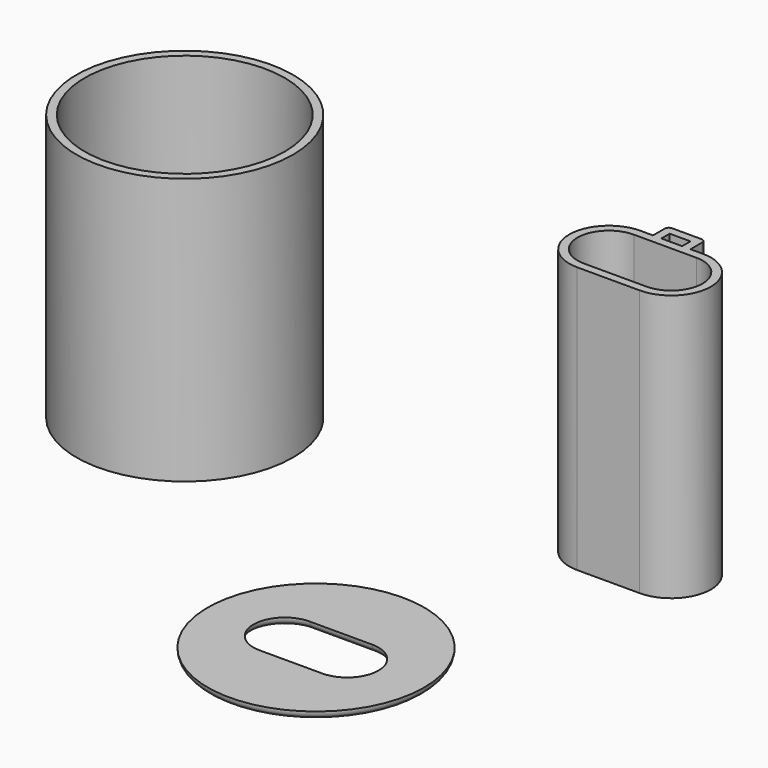
from build123d import *

# Parameters (mm, degrees)
F0_R         = 33.02
F0_R_2       = 30.48
F1_DEPTH     = 81.28
F2_DEPTH     = 2.54
F3_DEPTH     = 1.27
F4_T1_DEPTH  = 19.05
F4_T8_ANGLE  = 180
F4_T12_ANGLE = 180


# Not quite as in the source:
# - a fillet or chamfer that OpenCascade refuses, or shapes differently, is made with other operations: its cross-section is extruded or revolved along the edge and cut away or added


with BuildPart() as f1:
    # F0 (on Top) → F1 (new body)
    with BuildSketch(Plane.XY):
        with Locations((-97.8379249573, 24.8728301376)):
            Circle(F0_R)
        with Locations((-97.8379249573, 24.8728301376)):
            Circle(F0_R_2, mode=Mode.SUBTRACT)
    extrude(amount=F1_DEPTH)


with BuildPart() as f1b:
    # F0 (on Top) → F1, piece 2 (new body)
    with BuildSketch(Plane.XY):
        with BuildLine():
            Line((36.9737733483, 45.9476387101), (39.5137733483, 45.9476387101))
            Line((39.5137733483, 45.9476387101), (39.5137733483, 50.3926387101))
            ThreePointArc((39.5137733483, 50.3926387101), (39.1417989604, 51.2906643222), (38.2437733483, 51.6626387101))
            Line((38.2437733483, 51.6626387101), (29.3537733483, 51.6626387101))
            ThreePointArc((29.3537733483, 51.6626387101), (28.4557477362, 51.2906643222), (28.0837733483, 50.3926387101))
            Line((28.0837733483, 50.3926387101), (28.0837733483, 45.9476387101))
            Line((28.0837733483, 45.9476387101), (30.6237733483, 45.9476387101))
            Line((30.6237733483, 45.9476387101), (30.6237733483, 49.1226387101))
            Line((30.6237733483, 49.1226387101), (36.9737733483, 49.1226387101))
            Line((36.9737733483, 49.1226387101), (36.9737733483, 45.9476387101))
        make_face()
        with BuildLine():
            ThreePointArc((43.3237733483, 21.8176387101), (55.3887733483, 33.8826387101), (43.3237733483, 45.9476387101))
            Line((43.3237733483, 45.9476387101), (39.5137733483, 45.9476387101))
            Line((39.5137733483, 45.9476387101), (36.9737733483, 45.9476387101))
            Line((36.9737733483, 45.9476387101), (30.6237733483, 45.9476387101))
            Line((30.6237733483, 45.9476387101), (28.0837733483, 45.9476387101))
            Line((28.0837733483, 45.9476387101), (24.2737733483, 45.9476387101))
            ThreePointArc((24.2737733483, 45.9476387101), (12.2087733483, 33.8826387101), (24.2737733483, 21.8176387101))
            Line((24.2737733483, 21.8176387101), (43.3237733483, 21.8176387101))
        make_face()
        with BuildLine():
            ThreePointArc((24.2737733483, 24.3576387101), (14.7487733483, 33.8826387101), (24.2737733483, 43.4076387101))
            Line((24.2737733483, 43.4076387101), (43.3237733483, 43.4076387101))
            ThreePointArc((43.3237733483, 43.4076387101), (52.8487733483, 33.8826387101), (43.3237733483, 24.3576387101))
            Line((43.3237733483, 24.3576387101), (24.2737733483, 24.3576387101))
        make_face(mode=Mode.SUBTRACT)
    extrude(amount=F1_DEPTH)


with BuildPart() as f2:
    # F0 (on Top) → F2 (new body)
    with BuildSketch(Plane.XY):
        with BuildLine():
            Line((23.8957638139, -31.8045213862), (27.0388534563, -28.6614317439))
            ThreePointArc((27.0388534563, -28.6614317439), (-19.6584783733, -28.6614317439), (-19.6584783733, -75.3587635734))
            Line((-19.6584783733, -75.3587635734), (-16.5153887309, -72.215673931))
            ThreePointArc((-16.5153887309, -72.215673931), (-16.5153887309, -67.7255458705), (-12.0252606704, -67.7255458705))
            Line((-12.0252606704, -67.7255458705), (-5.8348124585, -61.5350976586))
            ThreePointArc((-5.8348124585, -61.5350976586), (-15.3598124585, -52.0100976586), (-5.8348124585, -42.4850976586))
            Line((-5.8348124585, -42.4850976586), (13.2151875415, -42.4850976586))
            Line((13.2151875415, -42.4850976586), (19.4056357534, -36.2946494468))
            ThreePointArc((19.4056357534, -36.2946494468), (19.4056357534, -31.8045213862), (23.8957638139, -31.8045213862))
        make_face()
        with BuildLine():
            ThreePointArc((-19.6584783733, -75.3587635734), (16.3263944782, -82.5165998222), (36.7101875415, -52.0100976586))
            ThreePointArc((36.7101875415, -52.0100976586), (34.196689705, -39.3738907219), (27.0388534563, -28.6614317439))
            Line((27.0388534563, -28.6614317439), (23.8957638139, -31.8045213862))
            ThreePointArc((23.8957638139, -31.8045213862), (24.5840172994, -32.8345655187), (24.8256997837, -34.0495854165))
            ThreePointArc((24.8256997837, -34.0495854165), (22.8657196814, -36.9829029322), (19.4056357534, -36.2946494468))
            Line((19.4056357534, -36.2946494468), (13.2151875415, -42.4850976586))
            ThreePointArc((13.2151875415, -42.4850976586), (22.7401875415, -52.0100976586), (13.2151875415, -61.5350976586))
            Line((13.2151875415, -61.5350976586), (-5.8348124585, -61.5350976586))
            Line((-5.8348124585, -61.5350976586), (-12.0252606704, -67.7255458705))
            ThreePointArc((-12.0252606704, -67.7255458705), (-11.3370071849, -68.755590003), (-11.0953247006, -69.9706099008))
            ThreePointArc((-11.0953247006, -69.9706099008), (-13.0553048029, -72.9039274165), (-16.5153887309, -72.215673931))
            Line((-16.5153887309, -72.215673931), (-19.6584783733, -75.3587635734))
        make_face()
        with BuildLine():
            Line((-14.2703247006, -69.9706099008), (-16.5153887309, -72.215673931))
            ThreePointArc((-16.5153887309, -72.215673931), (-13.0553048029, -72.9039274165), (-11.0953247006, -69.9706099008))
            ThreePointArc((-11.0953247006, -69.9706099008), (-11.3370071849, -68.755590003), (-12.0252606704, -67.7255458705))
            Line((-12.0252606704, -67.7255458705), (-14.2703247006, -69.9706099008))
        make_face()
        with BuildLine():
            ThreePointArc((-12.0252606704, -67.7255458705), (-16.5153887309, -67.7255458705), (-16.5153887309, -72.215673931))
            Line((-16.5153887309, -72.215673931), (-14.2703247006, -69.9706099008))
            Line((-14.2703247006, -69.9706099008), (-12.0252606704, -67.7255458705))
        make_face()
        with BuildLine():
            Line((21.6506997837, -34.0495854165), (23.8957638139, -31.8045213862))
            ThreePointArc((23.8957638139, -31.8045213862), (19.4056357534, -31.8045213862), (19.4056357534, -36.2946494468))
            Line((19.4056357534, -36.2946494468), (21.6506997837, -34.0495854165))
        make_face()
        with BuildLine():
            ThreePointArc((24.8256997837, -34.0495854165), (24.5840172994, -32.8345655187), (23.8957638139, -31.8045213862))
            Line((23.8957638139, -31.8045213862), (21.6506997837, -34.0495854165))
            Line((21.6506997837, -34.0495854165), (19.4056357534, -36.2946494468))
            ThreePointArc((19.4056357534, -36.2946494468), (22.8657196814, -36.9829029322), (24.8256997837, -34.0495854165))
        make_face()
    extrude(amount=F2_DEPTH)

    # F0 (on Top) → F3 (join)
    with BuildSketch(Plane.XY):
        with BuildLine():
            ThreePointArc((24.8256997837, -34.0495854165), (24.5840172994, -32.8345655187), (23.8957638139, -31.8045213862))
            Line((23.8957638139, -31.8045213862), (21.6506997837, -34.0495854165))
            Line((21.6506997837, -34.0495854165), (19.4056357534, -36.2946494468))
            ThreePointArc((19.4056357534, -36.2946494468), (22.8657196814, -36.9829029322), (24.8256997837, -34.0495854165))
        make_face()
        with BuildLine():
            Line((21.6506997837, -34.0495854165), (23.8957638139, -31.8045213862))
            ThreePointArc((23.8957638139, -31.8045213862), (19.4056357534, -31.8045213862), (19.4056357534, -36.2946494468))
            Line((19.4056357534, -36.2946494468), (21.6506997837, -34.0495854165))
        make_face()
        with BuildLine():
            ThreePointArc((-12.0252606704, -67.7255458705), (-16.5153887309, -67.7255458705), (-16.5153887309, -72.215673931))
            Line((-16.5153887309, -72.215673931), (-14.2703247006, -69.9706099008))
            Line((-14.2703247006, -69.9706099008), (-12.0252606704, -67.7255458705))
        make_face()
        with BuildLine():
            Line((-14.2703247006, -69.9706099008), (-16.5153887309, -72.215673931))
            ThreePointArc((-16.5153887309, -72.215673931), (-13.0553048029, -72.9039274165), (-11.0953247006, -69.9706099008))
            ThreePointArc((-11.0953247006, -69.9706099008), (-11.3370071849, -68.755590003), (-12.0252606704, -67.7255458705))
            Line((-12.0252606704, -67.7255458705), (-14.2703247006, -69.9706099008))
        make_face()
    extrude(amount=-F3_DEPTH)

    # F4: fillet of radius 2.54 on 7 edges, made by hand

    # F4_s2 → F4_t1 (cut)
    with BuildSketch(Plane.YZ.offset(-5.8348124585)):
        with BuildLine():
            ThreePointArc((-64.0750976586, 0), (-62.2790464344, 0.7439487758), (-61.5350976586, 2.54))
            Line((-61.5350976586, 2.54), (-61.5350976586, 0))
            Line((-61.5350976586, 0), (-64.0750976586, 0))
        make_face()
        with BuildLine():
            ThreePointArc((-39.9450976586, 0), (-41.7411488828, 0.7439487758), (-42.4850976586, 2.54))
            Line((-42.4850976586, 2.54), (-42.4850976586, 0))
            Line((-42.4850976586, 0), (-39.9450976586, 0))
        make_face()
    extrude(amount=F4_T1_DEPTH, mode=Mode.SUBTRACT)

    # F4_s3 → F4_t4 (revolve, cut)
    with BuildSketch(Plane.XZ.offset(34.0495854165)):
        with BuildLine():
            ThreePointArc((24.8256997837, 0), (23.895995258, -0.9297045256), (22.625995258, -1.27))
            Line((22.625995258, -1.27), (24.8256997837, -1.27))
            Line((24.8256997837, -1.27), (24.8256997837, 0))
        make_face()
    revolve(axis=Axis((21.6506997837, -34.0495854165, -1.27), (0, 0, 1)), mode=Mode.SUBTRACT)

    # F4_s5 → F4_t6 (revolve, cut)
    with BuildSketch(Plane(origin=(27.8501426001, -27.8501426001, 0), x_dir=(0, 0, 1), z_dir=(-0.7071067812, 0.7071067812, 0))):
        with BuildLine():
            ThreePointArc((0, -62.7423361101), (-0.9297045256, -61.8126315845), (-1.27, -60.5426315845))
            Line((-1.27, -60.5426315845), (-1.27, -62.7423361101))
            Line((-1.27, -62.7423361101), (0, -62.7423361101))
        make_face()
    revolve(axis=Axis((-14.2703247006, -69.9706099008, -1.27), (0, 0, 1)), mode=Mode.SUBTRACT)

    # F4_s7 → F4_t8 (revolve, cut)
    with BuildSketch(Plane.YZ.offset(13.2151875415)):
        with BuildLine():
            ThreePointArc((-39.9450976586, 0), (-41.7411488828, 0.7439487758), (-42.4850976586, 2.54))
            Line((-42.4850976586, 2.54), (-42.4850976586, 0))
            Line((-42.4850976586, 0), (-39.9450976586, 0))
        make_face()
    revolve(axis=Axis((13.2151875415, -52.0100976586, 0), (0, 0, -1)), revolution_arc=F4_T8_ANGLE, mode=Mode.SUBTRACT)

    # F4_s9 → F4_t10 (revolve, cut)
    with BuildSketch(Plane(origin=(27.8501426001, -27.8501426001, 0), x_dir=(0, 0, 1), z_dir=(-0.7071067812, 0.7071067812, 0))):
        with BuildLine():
            ThreePointArc((2.54, -67.1873361101), (0.7439487758, -66.4433873344), (0, -64.6473361101))
            Line((0, -64.6473361101), (0, -67.1873361101))
            Line((0, -67.1873361101), (2.54, -67.1873361101))
        make_face()
    revolve(axis=Axis((3.6901875415, -52.0100976586, 0), (0, 0, 1)), mode=Mode.SUBTRACT)

    # F4_s11 → F4_t12 (revolve, cut)
    with BuildSketch(Plane.YZ.offset(-5.8348124585)):
        with BuildLine():
            ThreePointArc((-64.0750976586, 0), (-62.2790464344, 0.7439487758), (-61.5350976586, 2.54))
            Line((-61.5350976586, 2.54), (-61.5350976586, 0))
            Line((-61.5350976586, 0), (-64.0750976586, 0))
        make_face()
    revolve(axis=Axis((-5.8348124585, -52.0100976586, 0), (0, 0, -1)), revolution_arc=F4_T12_ANGLE, mode=Mode.SUBTRACT)


solid = Compound([f1.part, f1b.part, f2.part])
